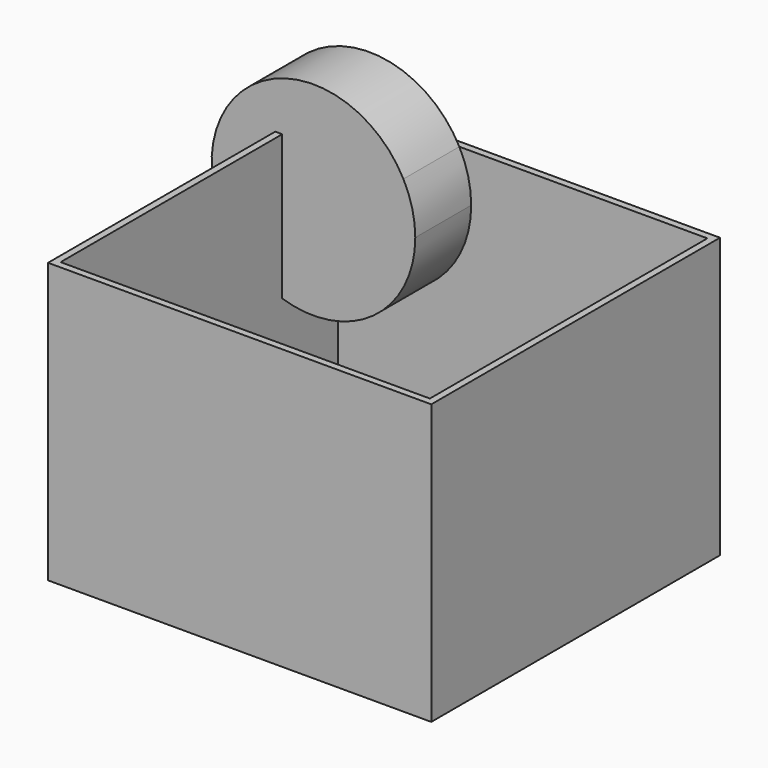
from build123d import *

# Parameters (mm, degrees)
F0_W     = 139.2736807466
F0_H     = 131.1470270157
F1_DEPTH = 101.6
F2_T     = -2.54
F4_DEPTH = 25.4


with BuildPart() as f1:
    # F0 (on Top) → F1 (new body)
    with BuildSketch(Plane.XY):
        with Locations((-2.6764906943, 1.5565976501)):
            Rectangle(F0_W, F0_H)
    extrude(amount=F1_DEPTH)

    # F2
    f2_openings = [f1.faces().sort_by_distance(p)[0] for p in [
        (-2.676491, 1.556598, 101.6),
    ]]
    offset(amount=F2_T, openings=f2_openings)

    # F3 (on face) → F4 (join)
    with BuildSketch(Plane.XZ.offset(-64.5901111579)):
        with BuildLine():
            Line((-69.7733310676, 101.6), (-25.7274541641, 101.6))
            ThreePointArc((-25.7274541641, 101.6), (-86.7891143722, 108.0409788687), (-69.7733310676, 49.0454224709))
            Line((-69.7733310676, 49.0454224709), (-69.7733310676, 101.6))
        make_face()
        with BuildLine():
            ThreePointArc((-69.7733310676, 49.0454224709), (-36.6361593712, 54.3579049697), (-21.4188937376, 84.2699334025))
            ThreePointArc((-21.4188937376, 84.2699334025), (-22.5121831898, 93.1987477306), (-25.7274541641, 101.6))
            Line((-25.7274541641, 101.6), (-69.7733310676, 101.6))
            Line((-69.7733310676, 101.6), (-69.7733310676, 49.0454224709))
        make_face()
    extrude(amount=F4_DEPTH)


solid = f1.part
